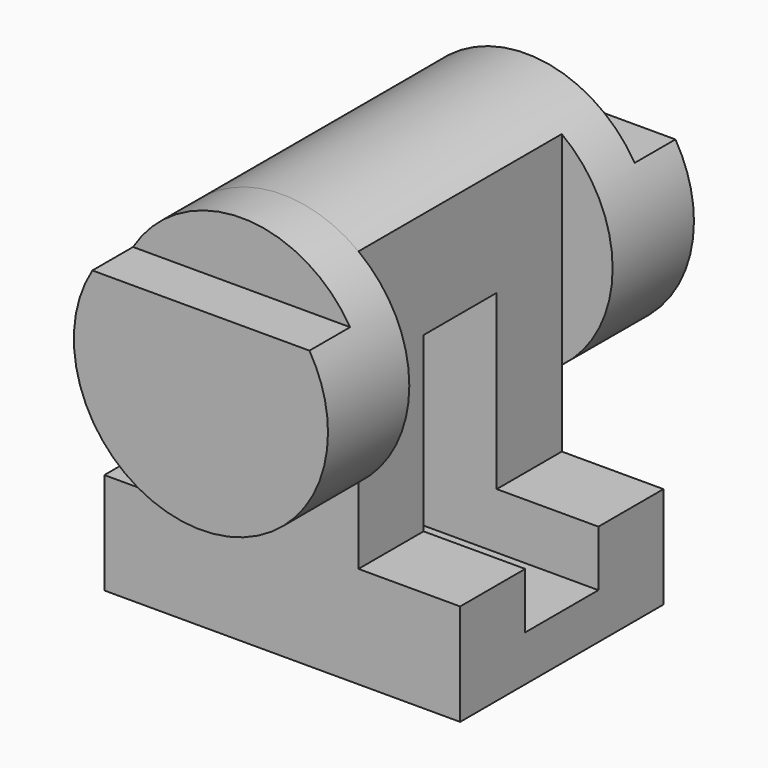
from build123d import *

# Parameters (mm, degrees)
F0_W          = 70
F0_H          = 50
F1_DEPTH      = 70
F2_R          = 25
F3_DEPTH      = 20
F3_DEPTH_BACK = 70
F4_W          = 18
F4_H          = 45
F5_DEPTH      = 70.001
F6_W          = 50
F6_H          = 20
F7_DEPTH      = 10
F8_W          = 50
F8_H          = 100
F9_DEPTH      = 20


# Not quite as in the source:
# - a pattern or mirror of a feature is missing from the dataset's text; its kind, count and spacing are read off the source's solid


with BuildPart() as f1:
    # F0 (on Top) → F1 (new body)
    with BuildSketch(Plane.XY):
        Rectangle(F0_W, F0_H)
    extrude(amount=F1_DEPTH)

    # F2 (on face) → F3 (join, two sides)
    with BuildSketch(Plane.XZ.offset(25)) as f3_sk:
        with Locations((0, 55)):
            Circle(F2_R)
    extrude(amount=F3_DEPTH)
    extrude(f3_sk.sketch, amount=-F3_DEPTH_BACK)

    # F4 (on face) → F5 (cut, through all)
    with BuildSketch(Plane.YZ.offset(35)):
        with Locations((0, 31.5)):
            Rectangle(F4_W, F4_H)
    extrude(amount=-F5_DEPTH, mode=Mode.SUBTRACT)

    # F6 (on face) → F7 (cut)
    with BuildSketch(Plane.XZ.offset(45)):
        with Locations((0, 78)):
            Rectangle(F6_W, F6_H)
    f7 = extrude(amount=-F7_DEPTH, mode=Mode.SUBTRACT)

    # F7_copies: F7 across plane
    add(f7.mirror(Plane.ZX), mode=Mode.SUBTRACT)

    # F8 (on face) → F9 (cut)
    with BuildSketch(Plane.YZ.offset(35)):
        with Locations((0, 70)):
            Rectangle(F8_W, F8_H)
    f9 = extrude(amount=-F9_DEPTH, mode=Mode.SUBTRACT)

    # F9_copies: F9 across plane
    add(f9.mirror(Plane(origin=(0, 0, 0), x_dir=(0, 0, -1), z_dir=(-1, 0, 0))), mode=Mode.SUBTRACT)


solid = f1.part
